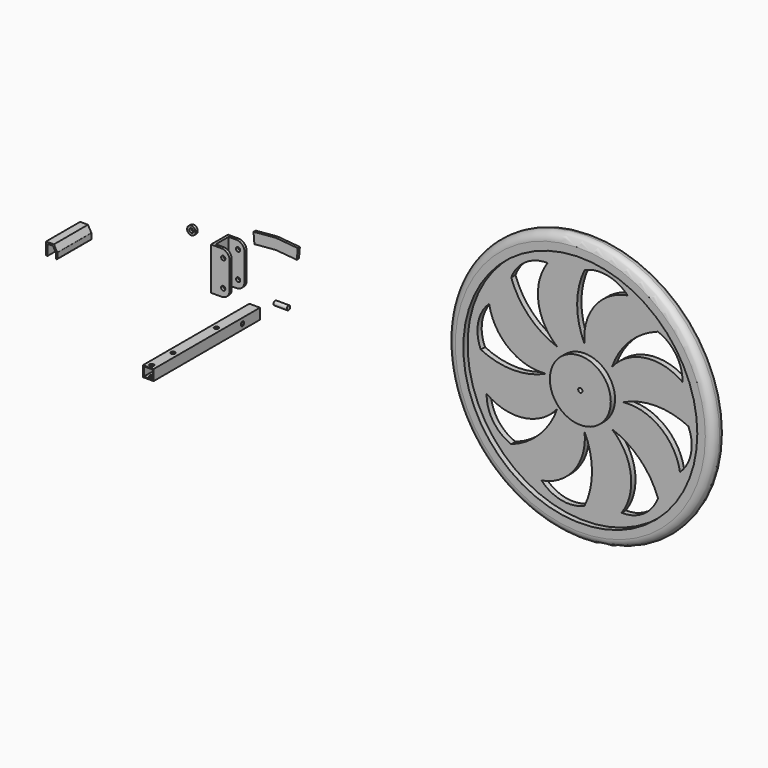
from build123d import *

# Parameters (mm, degrees)
F0_W         = 5
F0_H         = 80
F0_W_2       = 30
F0_R         = 4
F1_DEPTH     = 5
F2_DEPTH     = 15
F0_W_3       = 20
F0_H_2       = 20
F0_W_4       = 17
F0_H_3       = 17
F5_DEPTH     = 250
F0_R_2       = 250
F0_R_3       = 219.9372385263
F6_DEPTH     = 15
F0_R_4       = 57.2664650893
F7_DEPTH     = 5
F9_R         = 14.99999
F9_2_R       = 14.99999
F11_DEPTH    = 5
F0_R_5       = 8
F12_DEPTH    = 80
F13_T1_DEPTH = 80
F13_T3_DEPTH = 87.5
F13_T5_DEPTH = 81.9373487951
F15_D        = 8
F15_ON_F10_D = 8
F15_ON_F14_D = 8
F14_R        = 4
F16_DEPTH    = 25


# Not quite as in the source:
# - a fillet or chamfer that OpenCascade refuses, or shapes differently, is made with other operations: its cross-section is extruded or revolved along the edge and cut away or added
# - a fillet or chamfer is up to 0.001 mm smaller than in the source, because OpenCascade refuses the exact size


with BuildPart() as f1:
    # F0 (on Front) → F1 (new body)
    with BuildSketch(Plane.XZ):
        with Locations((-17.5, 0)):
            Rectangle(F0_W, F0_H)
        Rectangle(F0_W_2, F0_H)
        with Locations((3, -25)):
            Circle(F0_R, mode=Mode.SUBTRACT)
        with Locations((3, 25)):
            Circle(F0_R, mode=Mode.SUBTRACT)
    extrude(amount=F1_DEPTH)

    # F0 (on Front) → F2 (join)
    with BuildSketch(Plane.XZ):
        with Locations((-17.5, 0)):
            Rectangle(F0_W, F0_H)
    extrude(amount=-F2_DEPTH)

    # F3: F1 across face


with BuildPart() as f1_1:
    add(f1.part)
    add(f1.part.mirror(Plane(origin=(-17.5, 15, 0), x_dir=(1, 0, 0), z_dir=(0, 1, 0))))

    # F9 (radius 15 in the source; OpenCascade refuses exactly that, so slightly less here)
    f9_edges = [f1_1.edges().sort_by_distance(p)[0] for p in [
        (15, -2.5, 40),
        (15, 32.5, 40),
        (15, 32.5, -40),
        (15, -2.5, -40),
    ]]
    fillet(f9_edges, radius=F9_R)

    # F15 (through all)
    with Locations(Plane(origin=(-20, 0, 0), x_dir=(0, -1, 0), z_dir=(-1, 0, 0))):
        with Locations((-15, 0)):
            Hole(F15_D / 2)


with BuildPart() as f5:
    # F0 (on Front) → F5 (new body)
    with BuildSketch(Plane.XZ):
        with Locations((58.16140607, -47.9098314047)):
            Rectangle(F0_W_3, F0_H_2)
        with Locations((58.16140607, -47.9098314047)):
            Rectangle(F0_W_4, F0_H_3, mode=Mode.SUBTRACT)
    extrude(amount=F5_DEPTH)

    # F15 on F10 (through all)
    with Locations(Plane.XY.offset(-37.9098314047)):
        with Locations((58.16140607, -242), (58.16140607, -192), (58.16140607, -90)):
            Hole(F15_ON_F10_D / 2)

    # F15 on F14 (through all)
    with Locations(Plane.YZ.offset(68.16140607)):
        with Locations((-41.1763228476, -47.9098314047)):
            Hole(F15_ON_F14_D / 2)


with BuildPart() as f6:
    # F0 (on Front) → F6 (new body)
    with BuildSketch(Plane.XZ):
        with Locations((682.2916865349, 30.9796202928)):
            Circle(F0_R_2)
        with Locations((682.2916865349, 30.9796202928)):
            Circle(F0_R_3, mode=Mode.SUBTRACT)
    extrude(amount=F6_DEPTH)



with BuildPart() as f6b:
    # F0 (on Front) → F6, piece 2 (new body)
    with BuildSketch(Plane.XZ):
        with Locations((682.2916865349, 30.9796202928)):
            Circle(F0_R_4)
        with Locations((682.2916865349, 30.9796202928)):
            Circle(F0_R, mode=Mode.SUBTRACT)
    extrude(amount=F6_DEPTH)


with BuildPart() as f6_1:
    add(f6.part)

    add(f6b.part)  # F7 merges F6b
    # F0 (on Front) → F7 (join)
    with BuildSketch(Plane.XZ):
        with Locations((682.2916865349, 30.9796202928)):
            Circle(F0_R_3)
        with BuildLine():
            ThreePointArc((682.2916865349, -164.1104370356), (639.2805700509, -169.1574944329), (601.2696623802, -148.4065949917))
            ThreePointArc((601.2696623802, -148.4065949917), (662.9837980392, -111.1628179813), (682.2916865349, -41.7154356837))
            ThreePointArc((682.2916865349, -41.7154356837), (696.2558945086, -102.9129363596), (682.2916865349, -164.1104370356))
        make_face(mode=Mode.SUBTRACT)
        with BuildLine():
            ThreePointArc((544.3421840559, -106.9698821862), (510.359923413, -80.1252385646), (498.1552545506, -38.574366281))
            ThreePointArc((498.1552545506, -38.574366281), (568.1290656512, -55.8775228195), (630.8885194952, -20.4235467469))
            ThreePointArc((630.8885194952, -20.4235467469), (597.4895379277, -73.5709006187), (544.3421840559, -106.9698821862))
        make_face(mode=Mode.SUBTRACT)
        with BuildLine():
            ThreePointArc((820.2411890138, -106.9698821862), (793.3965453923, -140.9521428291), (751.8456731087, -153.1568116915))
            ThreePointArc((751.8456731087, -153.1568116915), (769.1488296472, -83.1830005909), (733.6948535746, -20.4235467469))
            ThreePointArc((733.6948535746, -20.4235467469), (786.8422074464, -53.8225283144), (820.2411890138, -106.9698821862))
        make_face(mode=Mode.SUBTRACT)
        with BuildLine():
            ThreePointArc((877.3817438632, 30.9796202928), (882.4288012606, -12.0314961912), (861.6779018193, -50.0424038619))
            ThreePointArc((861.6779018193, -50.0424038619), (824.4341248089, 11.6717317971), (754.9867425114, 30.9796202928))
            ThreePointArc((754.9867425114, 30.9796202928), (816.1842431873, 44.9438282665), (877.3817438632, 30.9796202928))
        make_face(mode=Mode.SUBTRACT)
        with BuildLine():
            ThreePointArc((487.2016292065, 30.9796202928), (482.1545718092, 73.9907367768), (502.9054712504, 112.0016444474))
            ThreePointArc((502.9054712504, 112.0016444474), (540.1492482608, 50.2875087884), (609.5966305584, 30.9796202928))
            ThreePointArc((609.5966305584, 30.9796202928), (548.3991298825, 17.015412319), (487.2016292065, 30.9796202928))
        make_face(mode=Mode.SUBTRACT)
        with BuildLine():
            ThreePointArc((544.3421840559, 168.9291227717), (571.1868276775, 202.9113834147), (612.7376999611, 215.116052277))
            ThreePointArc((612.7376999611, 215.116052277), (595.4345434226, 145.1422411764), (630.8885194952, 82.3827873325))
            ThreePointArc((630.8885194952, 82.3827873325), (577.7411656234, 115.7817689), (544.3421840559, 168.9291227717))
        make_face(mode=Mode.SUBTRACT)
        with Locations((682.2916865349, 30.9796202928)):
            Circle(F0_R_4, mode=Mode.SUBTRACT)
        with BuildLine():
            ThreePointArc((820.2411890138, 168.9291227717), (854.2234496568, 142.0844791502), (866.4281185191, 100.5336068666))
            ThreePointArc((866.4281185191, 100.5336068666), (796.4543074185, 117.8367634051), (733.6948535746, 82.3827873325))
            ThreePointArc((733.6948535746, 82.3827873325), (767.0938351421, 135.5301412043), (820.2411890138, 168.9291227717))
        make_face(mode=Mode.SUBTRACT)
        with BuildLine():
            ThreePointArc((682.2916865349, 226.0696776211), (725.3028030189, 231.1167350185), (763.3137106895, 210.3658355772))
            ThreePointArc((763.3137106895, 210.3658355772), (701.5995750305, 173.1220585668), (682.2916865349, 103.6746762693))
            ThreePointArc((682.2916865349, 103.6746762693), (668.3274785611, 164.8721769452), (682.2916865349, 226.0696776211))
        make_face(mode=Mode.SUBTRACT)
    extrude(amount=F7_DEPTH)

    # F8: F6 across face


with BuildPart() as f6_2:
    add(f6_1.part)
    add(f6_1.part.mirror(Plane(origin=(682.2916865349, 0, 30.9796202928), x_dir=(-1, 0, 0), z_dir=(0, 1, 0))))

    # F9#2 (radius 15 in the source; OpenCascade refuses exactly that, so slightly less here)
    f9_2_edges = [f6_2.edges().sort_by_distance(p)[0] for p in [
        (932.291687, -7.5, 30.97962),
        (432.291687, 0, 30.97962),
        (432.291687, -15, 30.97962),
        (932.291687, 7.5, 30.97962),
        (432.291687, 15, 30.97962),
    ]]
    fillet(f9_2_edges, radius=F9_2_R)


with BuildPart() as f11:
    # F0 (on Front) → F11 (new body)
    with BuildSketch(Plane.XZ):
        Polygon((59.9255195597, 86.9780315494), (61.6686344147, 67.0541375875), (101.5164223383, 70.5403672975), (141.364210262, 67.0541375875), (143.107325117, 86.9780315494), (103.2595371933, 90.4642612593), (99.7733074834, 90.4642612593), align=None)
    extrude(amount=F11_DEPTH)


with BuildPart() as f11b:
    # F0 (on Front) → F11, piece 2 (new body)
    with BuildSketch(Plane.XZ):
        with Locations((-56.8825379014, 51.0058514774)):
            Circle(F0_R_5)
        with Locations((-56.8825379014, 51.0058514774)):
            Circle(F0_R, mode=Mode.SUBTRACT)
    extrude(amount=F11_DEPTH)


with BuildPart() as f12:
    # F0 (on Front) → F12 (new body)
    with BuildSketch(Plane.XZ):
        Polygon((-266.989300251, -28.8267955184), (-266.989300251, -8.8267955184), (-256.989300251, -8.8267955184), (-251.4536678791, -18.8267955184), (-251.4536678791, -28.8638491184), (-248.8289791451, -28.8638491184), (-248.8289791451, -17.3738643262), (-255.2210119343, -5.8267955184), (-269.989300251, -5.8267955184), (-269.989300251, -28.8267955184), align=None)
    extrude(amount=F12_DEPTH)

    # F13: fillet of radius 1.5 on 5 edges, made by hand

    # F13_s2 → F13_t1 (join)
    with BuildSketch(Plane.XZ):
        with BuildLine():
            ThreePointArc((-251.6413235121, -18.4877996813), (-251.5013393091, -18.8391096767), (-251.4536678791, -19.2142652774))
            Line((-251.4536678791, -19.2142652774), (-251.4536678791, -18.8267955184))
            Line((-251.4536678791, -18.8267955184), (-251.6413235121, -18.4877996813))
        make_face()
        with BuildLine():
            ThreePointArc((-257.8734444093, -8.8267955184), (-257.1117680982, -9.0345690688), (-256.5611000423, -9.6003299223))
            Line((-256.5611000423, -9.6003299223), (-256.989300251, -8.8267955184))
            Line((-256.989300251, -8.8267955184), (-257.8734444093, -8.8267955184))
        make_face()
    extrude(amount=F13_T1_DEPTH)

    # F13_s4 → F13_t3 (cut)
    with BuildSketch(Plane.XZ.offset(-3.75)):
        with BuildLine():
            ThreePointArc((-249.9536678791, -28.8638491184), (-251.0143280509, -28.4245092901), (-251.4536678791, -27.3638491184))
            Line((-251.4536678791, -27.3638491184), (-251.4536678791, -28.8638491184))
            Line((-251.4536678791, -28.8638491184), (-249.9536678791, -28.8638491184))
        make_face()
        with BuildLine():
            ThreePointArc((-248.8289791451, -27.3638491184), (-249.2683189733, -28.4245092901), (-250.3289791451, -28.8638491184))
            Line((-250.3289791451, -28.8638491184), (-248.8289791451, -28.8638491184))
            Line((-248.8289791451, -28.8638491184), (-248.8289791451, -27.3638491184))
        make_face()
    extrude(amount=F13_T3_DEPTH, mode=Mode.SUBTRACT)

    # F13_s6 → F13_t5 (cut)
    with BuildSketch(Plane.XZ.offset(-0.9686743976)):
        with BuildLine():
            ThreePointArc((-249.016634778, -17.0348684891), (-248.876650575, -17.3861784845), (-248.8289791451, -17.7613340852))
            Line((-248.8289791451, -17.7613340852), (-248.8289791451, -17.3738643262))
            Line((-248.8289791451, -17.3738643262), (-249.016634778, -17.0348684891))
        make_face()
    extrude(amount=F13_T5_DEPTH, mode=Mode.SUBTRACT)


with BuildPart() as f16:
    # F14 (on face) → F16 (new body)
    with BuildSketch(Plane.YZ.offset(68.16140607)):
        with Locations((35.822533071, -44.7543822229)):
            Circle(F14_R)
    extrude(amount=F16_DEPTH)


solid = Compound([f1_1.part, f5.part, f6_2.part, f11.part, f11b.part, f12.part, f16.part])
